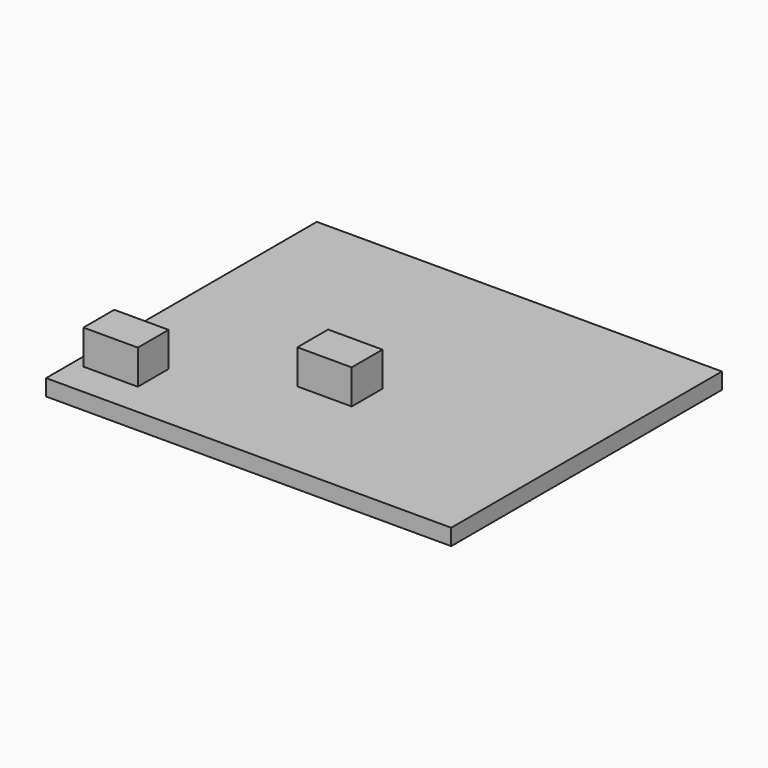
from build123d import *

# Parameters (mm, degrees)
F0_W     = 63.3566528559
F0_H     = 52.9265124351
F1_DEPTH = 2.54
F2_W     = 8.5002798587
F2_H     = 6.0210302472
F3_DEPTH = 7.9248


# Not quite as in the source:
# - the program builds the solid bodies; features that only make, move or delete a surface that nothing else refers to are left out


with BuildPart() as f1:
    # F0 (on Top) → F1 (new body)
    with BuildSketch(Plane.XY):
        with Locations((1.5970468521, -1.6539534554)):
            Rectangle(F0_W, F0_H)
    extrude(amount=F1_DEPTH)


with BuildPart() as f3:
    # F2 (on Top) → F3 (new body)
    with BuildSketch(Plane.XY):
        with Locations((-24.1524232551, -19.89361085)):
            Rectangle(F2_W, F2_H)
    extrude(amount=F3_DEPTH)


with BuildPart() as f3b:
    # F2 (on Top) → F3, piece 2 (new body)
    with BuildSketch(Plane.XY):
        with Locations((-0.4950552247, -7.6572103426)):
            Rectangle(F2_W, F2_H)
    extrude(amount=F3_DEPTH)


solid = Compound([f1.part, f3.part, f3b.part])
